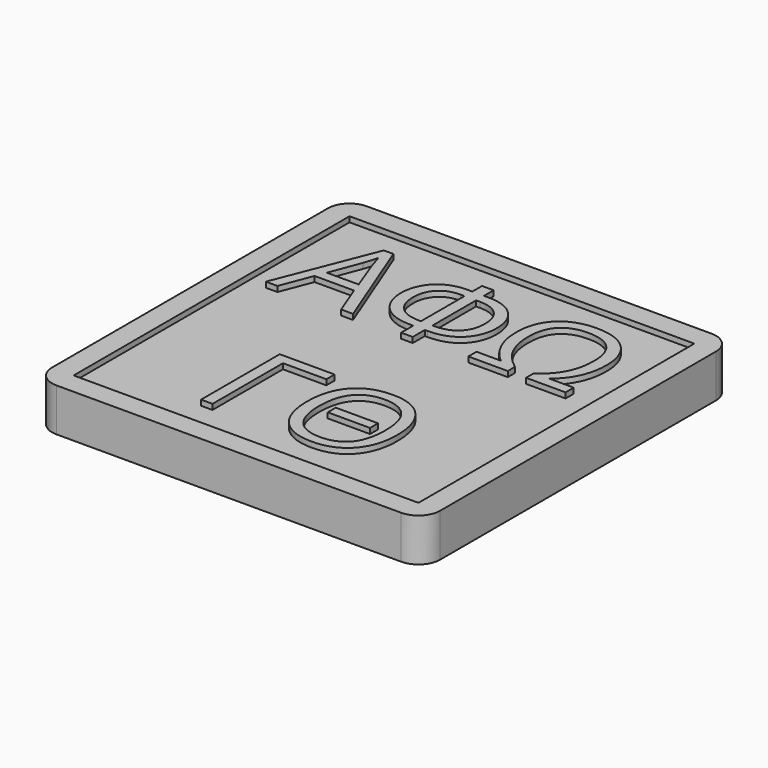
from build123d import *

# Parameters (mm, degrees)
F0_W         = 457.2
F0_H         = 457.2
F1_DEPTH     = 50.8
F2_R         = 25.4
F3_W         = 406.4
F3_H         = 406.4
F4_DEPTH     = 6.35
F5_TEXT_SIZE = 162.4012278499
F6_DEPTH     = 6.35


# Not quite as in the source:
# - Text() gives the source's letters only with a copy of the font that has no kerning and outlines rounded to 1/6400 em; it was checked with that copy


with BuildPart() as f1:
    # F0 (on Top) → F1 (new body)
    with BuildSketch(Plane.XY):
        Rectangle(F0_W, F0_H)
    extrude(amount=F1_DEPTH)

    # F2
    f2_edges = [f1.edges().sort_by_distance(p)[0] for p in [
        (-228.6, -228.6, 25.4),
        (228.6, -228.6, 25.4),
        (228.6, 228.6, 25.4),
        (-228.6, 228.6, 25.4),
    ]]
    fillet(f2_edges, radius=F2_R)

    # F3 (on face) → F4 (cut)
    with BuildSketch(Plane.XY.offset(50.8)):
        Rectangle(F3_W, F3_H)
    extrude(amount=-F4_DEPTH, mode=Mode.SUBTRACT)

    # F5 (on face) → F6 (join)
    with BuildSketch(Plane.XY.offset(44.45)):
        with Locations((-181.864, 53.2511159481)):
            Text('ΑΦΩ', F5_TEXT_SIZE, font='Open Sans', text_align=(TextAlign.LEFT, TextAlign.BOTTOM))
        with Locations((-97.4661119018, -167.6145539277)):
            Text('ΓΘ', F5_TEXT_SIZE, font='Open Sans', text_align=(TextAlign.LEFT, TextAlign.BOTTOM))
    extrude(amount=F6_DEPTH)


solid = f1.part
